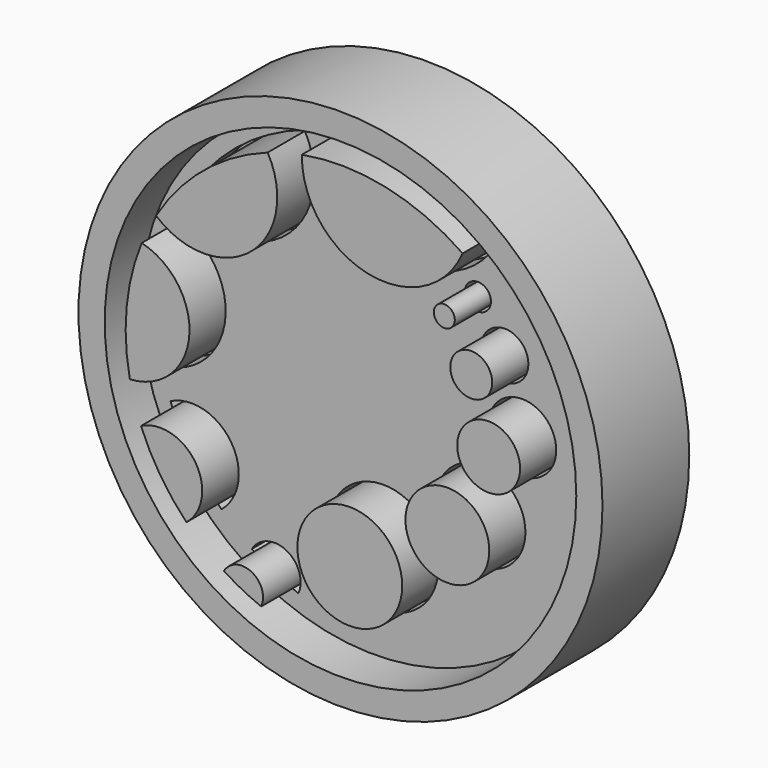
from build123d import *

# Parameters (mm, degrees)
F0_R         = 25
F0_R_2       = 22.5
F0_R_3       = 5
F0_R_4       = 4
F0_W         = 0.7168108311
F0_H         = 2.62805566
F0_R_5       = 2
F0_R_6       = 1
F0_R_7       = 3
F0_TEXT_SIZE = 4.8138397894
F2_DEPTH     = 4
F3_DEPTH     = 10.35
F4_DEPTH     = 10.35
F1_R         = 22.25
F1_R_2       = 5.25
F1_R_3       = 4.25
F1_W         = 0.7168108311
F1_H         = 2.62805566
F1_R_4       = 2.25
F1_R_5       = 1.25
F1_R_6       = 3.25
F1_TEXT_SIZE = 4.8138397894
F5_DEPTH     = 6.35


# Not quite as in the source:
# - Text() gives the source's letters only with a copy of the font that has no kerning and outlines rounded to 1/6400 em; it was checked with that copy


with BuildPart() as f2:
    # F0 (on Front) → F2 (new body)
    with BuildSketch(Plane.XZ):
        Circle(F0_R)
        Circle(F0_R_2, mode=Mode.SUBTRACT)
        Circle(F0_R_2)
        with BuildLine():
            ThreePointArc((11.6569283477, 16.8631557395), (18.1551236725, 9.5205821479), (20.5, 0))
            ThreePointArc((20.5, 0), (11.5132317321, -16.9615888136), (-7.5678531789, -19.0519709811))
            ThreePointArc((-7.5678531789, -19.0519709811), (-9.3883533238, -18.2238531016), (-11.1194937702, -17.2222779647))
            ThreePointArc((-11.1194937702, -17.2222779647), (-12.9920933667, -15.857348768), (-14.698689069, -14.2898054449))
            ThreePointArc((-14.698689069, -14.2898054449), (-17.1938340813, -11.1634255309), (-19.0343655416, -7.6120252515))
            ThreePointArc((-19.0343655416, -7.6120252515), (-19.6480708819, -5.8483596522), (-20.098740453, -4.0361655322))
            ThreePointArc((-20.098740453, -4.0361655322), (-20.406477126, 1.9559374492), (-18.9661277157, 7.7804883827))
            ThreePointArc((-18.9661277157, 7.7804883827), (-18.3325719196, 9.1742469344), (-17.5967657031, 10.5168358734))
            ThreePointArc((-17.5967657031, 10.5168358734), (-13.0325099947, 15.8241487366), (-6.9486992839, 19.2864091594))
            ThreePointArc((-6.9486992839, 19.2864091594), (-5.3345009161, 19.7937641689), (-3.6839600887, 20.1662698104))
            ThreePointArc((-3.6839600887, 20.1662698104), (4.315054618, 20.040716146), (11.6569283477, 16.8631557395))
        make_face(mode=Mode.SUBTRACT)
        with BuildLine():
            ThreePointArc((-7.5678531789, -19.0519709811), (11.5132317321, -16.9615888136), (20.5, 0))
            ThreePointArc((20.5, 0), (18.1551236725, 9.5205821479), (11.6569283477, 16.8631557395))
            ThreePointArc((11.6569283477, 16.8631557395), (2.6311308646, 12.2199488695), (-3.6839600887, 20.1662698104))
            ThreePointArc((-3.6839600887, 20.1662698104), (-5.3345009161, 19.7937641689), (-6.9486992839, 19.2864091594))
            ThreePointArc((-6.9486992839, 19.2864091594), (-8.5823846306, 10.4207808753), (-17.5967657031, 10.5168358734))
            ThreePointArc((-17.5967657031, 10.5168358734), (-18.3325719196, 9.1742469344), (-18.9661277157, 7.7804883827))
            ThreePointArc((-18.9661277157, 7.7804883827), (-14.4338496745, 1.3834679519), (-20.098740453, -4.0361655322))
            ThreePointArc((-20.098740453, -4.0361655322), (-19.6480708819, -5.8483596522), (-19.0343655416, -7.6120252515))
            ThreePointArc((-19.0343655416, -7.6120252515), (-13.8389396265, -8.985196159), (-14.698689069, -14.2898054449))
            ThreePointArc((-14.698689069, -14.2898054449), (-12.9920933667, -15.857348768), (-11.1194937702, -17.2222779647))
            ThreePointArc((-11.1194937702, -17.2222779647), (-8.4724164141, -16.4459162136), (-7.5678531789, -19.0519709811))
        make_face()
        with BuildLine():
            add(Edge.make_bspline(
                [(-3.0782241477, -4.3214418661), (-2.8995855618, -4.5527318248), (-2.8995855618, -4.8889484475)],
                knots=[0, 0, 0, 1, 1, 1], degree=2))
            add(Edge.make_bspline(
                [(-2.8995855618, -4.8889484475), (-2.8995855618, -5.3545370147), (-3.2346739408, -5.6226829342)],
                knots=[0, 0, 0, 1, 1, 1], degree=2))
            add(Edge.make_bspline(
                [(-3.2346739408, -5.6226829342), (-3.5697623199, -5.8908288537), (-4.1662271563, -5.8908288537)],
                knots=[0, 0, 0, 1, 1, 1], degree=2))
            add(Edge.make_bspline(
                [(-4.1662271563, -5.8908288537), (-4.7168100823, -5.8908288537), (-5.1395253888, -5.6832320128)],
                knots=[0, 0, 0, 1, 1, 1], degree=2))
            Line((-5.1395253888, -5.6832320128), (-5.1395253888, -5.0062857924))
            add(Edge.make_bspline(
                [(-5.1395253888, -5.0062857924), (-4.792026329, -5.1619834231), (-4.5509582583, -5.2251650703)],
                knots=[0, 0, 0, 1, 1, 1], degree=2))
            add(Edge.make_bspline(
                [(-4.5509582583, -5.2251650703), (-4.3098901876, -5.2883467176), (-4.1098149713, -5.2883467176)],
                knots=[0, 0, 0, 1, 1, 1], degree=2))
            add(Edge.make_bspline(
                [(-4.1098149713, -5.2883467176), (-3.8706273068, -5.2883467176), (-3.7423836061, -5.1969589778)],
                knots=[0, 0, 0, 1, 1, 1], degree=2))
            add(Edge.make_bspline(
                [(-3.7423836061, -5.1969589778), (-3.6141399055, -5.1055712381), (-3.6141399055, -4.9243000835)],
                knots=[0, 0, 0, 1, 1, 1], degree=2))
            add(Edge.make_bspline(
                [(-3.6141399055, -4.9243000835), (-3.6141399055, -4.8235103129), (-3.6705520905, -4.7445332539)],
                knots=[0, 0, 0, 1, 1, 1], degree=2))
            add(Edge.make_bspline(
                [(-3.6705520905, -4.7445332539), (-3.7269642756, -4.6655561948), (-3.8364039145, -4.5929725167)],
                knots=[0, 0, 0, 1, 1, 1], degree=2))
            add(Edge.make_bspline(
                [(-3.8364039145, -4.5929725167), (-3.9458435535, -4.5203888387), (-4.2820601763, -4.3601782332)],
                knots=[0, 0, 0, 1, 1, 1], degree=2))
            add(Edge.make_bspline(
                [(-4.2820601763, -4.3601782332), (-4.5964640875, -4.2120022272), (-4.7540421244, -4.0758608206)],
                knots=[0, 0, 0, 1, 1, 1], degree=2))
            add(Edge.make_bspline(
                [(-4.7540421244, -4.0758608206), (-4.9116201612, -3.9397194141), (-5.0056404696, -3.7584482595)],
                knots=[0, 0, 0, 1, 1, 1], degree=2))
            add(Edge.make_bspline(
                [(-5.0056404696, -3.7584482595), (-5.099660778, -3.5771771049), (-5.099660778, -3.335732953)],
                knots=[0, 0, 0, 1, 1, 1], degree=2))
            add(Edge.make_bspline(
                [(-5.099660778, -3.335732953), (-5.099660778, -2.8791703355), (-4.790522004, -2.6185460406)],
                knots=[0, 0, 0, 1, 1, 1], degree=2))
            add(Edge.make_bspline(
                [(-4.790522004, -2.6185460406), (-4.4813832301, -2.3579217458), (-3.9360654414, -2.3579217458)],
                knots=[0, 0, 0, 1, 1, 1], degree=2))
            add(Edge.make_bspline(
                [(-3.9360654414, -2.3579217458), (-3.6682956031, -2.3579217458), (-3.424971045, -2.421103393)],
                knots=[0, 0, 0, 1, 1, 1], degree=2))
            add(Edge.make_bspline(
                [(-3.424971045, -2.421103393), (-3.1816464869, -2.4842850402), (-2.916133136, -2.5993658977)],
                knots=[0, 0, 0, 1, 1, 1], degree=2))
            Line((-2.916133136, -2.5993658977), (-3.1508078258, -3.1664963979))
            add(Edge.make_bspline(
                [(-3.1508078258, -3.1664963979), (-3.4260992887, -3.0536720278), (-3.6058661184, -3.008918361)],
                knots=[0, 0, 0, 1, 1, 1], degree=2))
            add(Edge.make_bspline(
                [(-3.6058661184, -3.008918361), (-3.785632948, -2.9641646943), (-3.9593824779, -2.9641646943)],
                knots=[0, 0, 0, 1, 1, 1], degree=2))
            add(Edge.make_bspline(
                [(-3.9593824779, -2.9641646943), (-4.1662271563, -2.9641646943), (-4.276795039, -3.06044149)],
                knots=[0, 0, 0, 1, 1, 1], degree=2))
            add(Edge.make_bspline(
                [(-4.276795039, -3.06044149), (-4.3873629217, -3.1567182858), (-4.3873629217, -3.311663754)],
                knots=[0, 0, 0, 1, 1, 1], degree=2))
            add(Edge.make_bspline(
                [(-4.3873629217, -3.311663754), (-4.3873629217, -3.4079405498), (-4.3426092549, -3.4797720654)],
                knots=[0, 0, 0, 1, 1, 1], degree=2))
            add(Edge.make_bspline(
                [(-4.3426092549, -3.4797720654), (-4.2978555881, -3.5516035811), (-4.2004505486, -3.6185460406)],
                knots=[0, 0, 0, 1, 1, 1], degree=2))
            add(Edge.make_bspline(
                [(-4.2004505486, -3.6185460406), (-4.1030455091, -3.6854885002), (-3.738998875, -3.8592380301)],
                knots=[0, 0, 0, 1, 1, 1], degree=2))
            add(Edge.make_bspline(
                [(-3.738998875, -3.8592380301), (-3.2568627336, -4.0901519075), (-3.0782241477, -4.3214418661)],
                knots=[0, 0, 0, 1, 1, 1], degree=2))
        make_face(mode=Mode.SUBTRACT)
        with BuildLine():
            Line((-0.1541925569, -5.8434426183), (-0.8221128276, -5.8434426183))
            Line((-0.8221128276, -5.8434426183), (-1.6494915414, -3.1476923362))
            Line((-1.6494915414, -3.1476923362), (-1.6705520905, -3.1476923362))
            add(Edge.make_bspline(
                [(-1.6705520905, -3.1476923362), (-1.6254223425, -3.9698059128), (-1.6254223425, -4.2450973757)],
                knots=[0, 0, 0, 1, 1, 1], degree=2))
            Line((-1.6254223425, -4.2450973757), (-1.6254223425, -5.8434426183))
            Line((-1.6254223425, -5.8434426183), (-2.276795039, -5.8434426183))
            Line((-2.276795039, -5.8434426183), (-2.276795039, -2.4068123061))
            Line((-2.276795039, -2.4068123061), (-1.2846927449, -2.4068123061))
            Line((-1.2846927449, -2.4068123061), (-0.471605118, -5.0348679662))
            Line((-0.471605118, -5.0348679662), (-0.4573140311, -5.0348679662))
            Line((-0.4573140311, -5.0348679662), (0.4054163187, -2.4068123061))
            Line((0.4054163187, -2.4068123061), (1.3967664503, -2.4068123061))
            Line((1.3967664503, -2.4068123061), (1.3967664503, -5.8434426183))
            Line((1.3967664503, -5.8434426183), (0.7175637425, -5.8434426183))
            Line((0.7175637425, -5.8434426183), (0.7175637425, -4.216515202))
            add(Edge.make_bspline(
                [(0.7175637425, -4.216515202), (0.7175637425, -4.1014343445), (0.7213245548, -3.9510018511)],
                knots=[0, 0, 0, 1, 1, 1], degree=2))
            add(Edge.make_bspline(
                [(0.7213245548, -3.9510018511), (0.7250853672, -3.8005693577), (0.7529153784, -3.152205311)],
                knots=[0, 0, 0, 1, 1, 1], degree=2))
            Line((0.7529153784, -3.152205311), (0.7318548294, -3.152205311))
            Line((0.7318548294, -3.152205311), (-0.1541925569, -5.8434426183))
        make_face(mode=Mode.SUBTRACT)
        with Locations((0.8882983216, -12.9391586339)):
            Circle(F0_R_3, mode=Mode.SUBTRACT)
        with Locations((10.1970146039, -7.2864832287)):
            Circle(F0_R_4, mode=Mode.SUBTRACT)
        with BuildLine():
            Line((-9.9315524666, 0.7033794953), (-9.9315524666, 4.1400098074))
            Line((-9.9315524666, 4.1400098074), (-8.8619774384, 4.1400098074))
            add(Edge.make_bspline(
                [(-8.8619774384, 4.1400098074), (-8.1308755204, 4.1400098074), (-7.8006761973, 3.9320368853)],
                knots=[0, 0, 0, 1, 1, 1], degree=2))
            add(Edge.make_bspline(
                [(-7.8006761973, 3.9320368853), (-7.4704768743, 3.7240639631), (-7.4704768743, 3.2705099955)],
                knots=[0, 0, 0, 1, 1, 1], degree=2))
            add(Edge.make_bspline(
                [(-7.4704768743, 3.2705099955), (-7.4704768743, 2.962123384), (-7.614892068, 2.7646807364)],
                knots=[0, 0, 0, 1, 1, 1], degree=2))
            add(Edge.make_bspline(
                [(-7.614892068, 2.7646807364), (-7.7593072616, 2.5672380887), (-7.9992470886, 2.527373478)],
                knots=[0, 0, 0, 1, 1, 1], degree=2))
            Line((-7.9992470886, 2.527373478), (-7.9992470886, 2.5040564415))
            add(Edge.make_bspline(
                [(-7.9992470886, 2.5040564415), (-7.6728085779, 2.4310966822), (-7.528017303, 2.2313975472)],
                knots=[0, 0, 0, 1, 1, 1], degree=2))
            add(Edge.make_bspline(
                [(-7.528017303, 2.2313975472), (-7.3832260281, 2.0316984122), (-7.3832260281, 1.6999947642)],
                knots=[0, 0, 0, 1, 1, 1], degree=2))
            add(Edge.make_bspline(
                [(-7.3832260281, 1.6999947642), (-7.3832260281, 1.2298932223), (-7.7232034632, 0.9666363588)],
                knots=[0, 0, 0, 1, 1, 1], degree=2))
            add(Edge.make_bspline(
                [(-7.7232034632, 0.9666363588), (-8.0631808983, 0.7033794953), (-8.6461068103, 0.7033794953)],
                knots=[0, 0, 0, 1, 1, 1], degree=2))
            Line((-8.6461068103, 0.7033794953), (-9.9315524666, 0.7033794953))
        make_face(mode=Mode.SUBTRACT)
        with Locations((-6.3952606276, 2.0174073253)):
            Rectangle(F0_W, F0_H, mode=Mode.SUBTRACT)
        with BuildLine():
            add(Edge.make_bspline(
                [(-6.3941323839, 3.657873666), (-6.7845047043, 3.657873666), (-6.7845047043, 4.0106378631)],
                knots=[0, 0, 0, 1, 1, 1], degree=2))
            add(Edge.make_bspline(
                [(-6.7845047043, 4.0106378631), (-6.7845047043, 4.3611455728), (-6.3941323839, 4.3611455728)],
                knots=[0, 0, 0, 1, 1, 1], degree=2))
            add(Edge.make_bspline(
                [(-6.3941323839, 4.3611455728), (-6.0037600634, 4.3611455728), (-6.0037600634, 4.0106378631)],
                knots=[0, 0, 0, 1, 1, 1], degree=2))
            add(Edge.make_bspline(
                [(-6.0037600634, 4.0106378631), (-6.0037600634, 3.8436577954), (-6.1011651029, 3.7507657307)],
                knots=[0, 0, 0, 1, 1, 1], degree=2))
            add(Edge.make_bspline(
                [(-6.1011651029, 3.7507657307), (-6.1985701424, 3.657873666), (-6.3941323839, 3.657873666)],
                knots=[0, 0, 0, 1, 1, 1], degree=2))
        make_face(mode=Mode.SUBTRACT)
        with BuildLine():
            add(Edge.make_bspline(
                [(-3.0515223801, 2.7436201873), (-2.8965769119, 2.435609657), (-2.8965769119, 2.0219203001)],
                knots=[0, 0, 0, 1, 1, 1], degree=2))
            add(Edge.make_bspline(
                [(-2.8965769119, 2.0219203001), (-2.8965769119, 1.3803257157), (-3.2350500221, 1.0181594878)],
                knots=[0, 0, 0, 1, 1, 1], degree=2))
            add(Edge.make_bspline(
                [(-3.2350500221, 1.0181594878), (-3.5735231323, 0.6559932599), (-4.1775095933, 0.6559932599)],
                knots=[0, 0, 0, 1, 1, 1], degree=2))
            add(Edge.make_bspline(
                [(-4.1775095933, 0.6559932599), (-4.5558473143, 0.6559932599), (-4.8450537829, 0.8218450839)],
                knots=[0, 0, 0, 1, 1, 1], degree=2))
            add(Edge.make_bspline(
                [(-4.8450537829, 0.8218450839), (-5.1342602515, 0.9876969079), (-5.2892057197, 1.2979639255)],
                knots=[0, 0, 0, 1, 1, 1], degree=2))
            add(Edge.make_bspline(
                [(-5.2892057197, 1.2979639255), (-5.4441511879, 1.6082309432), (-5.4441511879, 2.0219203001)],
                knots=[0, 0, 0, 1, 1, 1], degree=2))
            add(Edge.make_bspline(
                [(-5.4441511879, 2.0219203001), (-5.4441511879, 2.6657713719), (-5.1083106464, 3.0230485438)],
                knots=[0, 0, 0, 1, 1, 1], degree=2))
            add(Edge.make_bspline(
                [(-5.1083106464, 3.0230485438), (-4.7724701048, 3.3803257157), (-4.1632185065, 3.3803257157)],
                knots=[0, 0, 0, 1, 1, 1], degree=2))
            add(Edge.make_bspline(
                [(-4.1632185065, 3.3803257157), (-3.7848807855, 3.3803257157), (-3.4956743169, 3.2159782166)],
                knots=[0, 0, 0, 1, 1, 1], degree=2))
            add(Edge.make_bspline(
                [(-3.4956743169, 3.2159782166), (-3.2064678483, 3.0516307176), (-3.0515223801, 2.7436201873)],
                knots=[0, 0, 0, 1, 1, 1], degree=2))
        make_face(mode=Mode.SUBTRACT)
        Polygon((-0.2685212519, 1.305109469), (-0.2685212519, 0.7033794953), (-2.2474607028, 0.7033794953), (-2.2474607028, 4.1400098074), (-0.2685212519, 4.1400098074), (-0.2685212519, 3.5427928086), (-1.5186152722, 3.5427928086), (-1.5186152722, 2.7883738541), (-0.3550199356, 2.7883738541), (-0.3550199356, 2.1911568552), (-1.5186152722, 2.1911568552), (-1.5186152722, 1.305109469), align=None, mode=Mode.SUBTRACT)
        with BuildLine():
            Line((3.2553599065, 4.1400098074), (3.2553599065, 0.7033794953))
            Line((3.2553599065, 0.7033794953), (2.5287709633, 0.7033794953))
            Line((2.5287709633, 0.7033794953), (2.5287709633, 2.6920970583))
            Line((2.5287709633, 2.6920970583), (2.5362925879, 3.018535569))
            Line((2.5362925879, 3.018535569), (2.5475750249, 3.3758127409))
            add(Edge.make_bspline(
                [(2.5475750249, 3.3758127409), (2.3670560328, 3.1952937488), (2.2963527609, 3.1388815637)],
                knots=[0, 0, 0, 1, 1, 1], degree=2))
            Line((2.2963527609, 3.1388815637), (1.9014674657, 2.8214690026))
            Line((1.9014674657, 2.8214690026), (1.550959756, 3.258475396))
            Line((1.550959756, 3.258475396), (2.6581429076, 4.1400098074))
            Line((2.6581429076, 4.1400098074), (3.2553599065, 4.1400098074))
        make_face(mode=Mode.SUBTRACT)
        with BuildLine():
            Line((6.6092523472, 1.314887581), (6.6092523472, 0.7033794953))
            Line((6.6092523472, 0.7033794953), (4.2068454273, 0.7033794953))
            Line((4.2068454273, 0.7033794953), (4.2068454273, 1.2088326732))
            Line((4.2068454273, 1.2088326732), (5.0695757771, 2.0805889725))
            add(Edge.make_bspline(
                [(5.0695757771, 2.0805889725), (5.4531786353, 2.4732177804), (5.5705159802, 2.6247785175)],
                knots=[0, 0, 0, 1, 1, 1], degree=2))
            add(Edge.make_bspline(
                [(5.5705159802, 2.6247785175), (5.687853325, 2.7763392546), (5.7397525353, 2.9057111989)],
                knots=[0, 0, 0, 1, 1, 1], degree=2))
            add(Edge.make_bspline(
                [(5.7397525353, 2.9057111989), (5.7916517455, 3.0350831433), (5.7916517455, 3.1734810372)],
                knots=[0, 0, 0, 1, 1, 1], degree=2))
            add(Edge.make_bspline(
                [(5.7916517455, 3.1734810372), (5.7916517455, 3.3803257157), (5.6773230505, 3.4814915675)],
                knots=[0, 0, 0, 1, 1, 1], degree=2))
            add(Edge.make_bspline(
                [(5.6773230505, 3.4814915675), (5.5629943555, 3.5826574193), (5.3726972513, 3.5826574193)],
                knots=[0, 0, 0, 1, 1, 1], degree=2))
            add(Edge.make_bspline(
                [(5.3726972513, 3.5826574193), (5.1733741976, 3.5826574193), (4.9853335808, 3.4908935983)],
                knots=[0, 0, 0, 1, 1, 1], degree=2))
            add(Edge.make_bspline(
                [(4.9853335808, 3.4908935983), (4.797292964, 3.3991297774), (4.592704773, 3.2298932223)],
                knots=[0, 0, 0, 1, 1, 1], degree=2))
            Line((4.592704773, 3.2298932223), (4.1978194777, 3.6977382768))
            add(Edge.make_bspline(
                [(4.1978194777, 3.6977382768), (4.4512982291, 3.9143610673), (4.6182782968, 4.0034923197)],
                knots=[0, 0, 0, 1, 1, 1], degree=2))
            add(Edge.make_bspline(
                [(4.6182782968, 4.0034923197), (4.7852583645, 4.092623572), (4.9827010121, 4.1407619699)],
                knots=[0, 0, 0, 1, 1, 1], degree=2))
            add(Edge.make_bspline(
                [(4.9827010121, 4.1407619699), (5.1801436598, 4.1889003678), (5.4245964616, 4.1889003678)],
                knots=[0, 0, 0, 1, 1, 1], degree=2))
            add(Edge.make_bspline(
                [(5.4245964616, 4.1889003678), (5.7465219975, 4.1889003678), (5.9932312867, 4.0715630229)],
                knots=[0, 0, 0, 1, 1, 1], degree=2))
            add(Edge.make_bspline(
                [(5.9932312867, 4.0715630229), (6.2399405759, 3.9542256781), (6.3764580637, 3.7424919436)],
                knots=[0, 0, 0, 1, 1, 1], degree=2))
            add(Edge.make_bspline(
                [(6.3764580637, 3.7424919436), (6.5129755514, 3.5307582091), (6.5129755514, 3.258475396)],
                knots=[0, 0, 0, 1, 1, 1], degree=2))
            add(Edge.make_bspline(
                [(6.5129755514, 3.258475396), (6.5129755514, 3.0207920564), (6.4294855176, 2.8128191343)],
                knots=[0, 0, 0, 1, 1, 1], degree=2))
            add(Edge.make_bspline(
                [(6.4294855176, 2.8128191343), (6.3459954838, 2.6048462121), (6.1707416289, 2.3863430154)],
                knots=[0, 0, 0, 1, 1, 1], degree=2))
            add(Edge.make_bspline(
                [(6.1707416289, 2.3863430154), (5.9954877741, 2.1678398187), (5.5539684059, 1.7631764114)],
                knots=[0, 0, 0, 1, 1, 1], degree=2))
            Line((5.5539684059, 1.7631764114), (5.1116968753, 1.3472305671))
            Line((5.1116968753, 1.3472305671), (5.1116968753, 1.314887581))
            Line((5.1116968753, 1.314887581), (6.6092523472, 1.314887581))
        make_face(mode=Mode.SUBTRACT)
        with BuildLine():
            add(Edge.make_bspline(
                [(8.9138781464, 3.9726536585), (9.2230169204, 3.7564069492), (9.2230169204, 3.3712997661)],
                knots=[0, 0, 0, 1, 1, 1], degree=2))
            add(Edge.make_bspline(
                [(9.2230169204, 3.3712997661), (9.2230169204, 3.0493742302), (9.0278307602, 2.82372549)],
                knots=[0, 0, 0, 1, 1, 1], degree=2))
            add(Edge.make_bspline(
                [(9.0278307602, 2.82372549), (8.8326446, 2.5980767499), (8.4798804029, 2.5130823911)],
                knots=[0, 0, 0, 1, 1, 1], degree=2))
            Line((8.4798804029, 2.5130823911), (8.4798804029, 2.4995434667))
            add(Edge.make_bspline(
                [(8.4798804029, 2.4995434667), (8.8965784097, 2.4476442565), (9.1101925503, 2.2464407965)],
                knots=[0, 0, 0, 1, 1, 1], degree=2))
            add(Edge.make_bspline(
                [(9.1101925503, 2.2464407965), (9.323806691, 2.0452373366), (9.323806691, 1.704507739)],
                knots=[0, 0, 0, 1, 1, 1], degree=2))
            add(Edge.make_bspline(
                [(9.323806691, 1.704507739), (9.323806691, 1.2088326732), (8.9642730317, 0.9324129665)],
                knots=[0, 0, 0, 1, 1, 1], degree=2))
            add(Edge.make_bspline(
                [(8.9642730317, 0.9324129665), (8.6047393724, 0.6559932599), (7.9375712641, 0.6559932599)],
                knots=[0, 0, 0, 1, 1, 1], degree=2))
            add(Edge.make_bspline(
                [(7.9375712641, 0.6559932599), (7.3779623886, 0.6559932599), (6.94546897, 0.8417773892)],
                knots=[0, 0, 0, 1, 1, 1], degree=2))
            Line((6.94546897, 0.8417773892), (6.94546897, 1.4600549372))
            add(Edge.make_bspline(
                [(6.94546897, 1.4600549372), (7.1447920238, 1.3592651666), (7.3847318508, 1.2957074381)],
                knots=[0, 0, 0, 1, 1, 1], degree=2))
            add(Edge.make_bspline(
                [(7.3847318508, 1.2957074381), (7.6246716778, 1.2321497097), (7.8593463675, 1.2321497097)],
                knots=[0, 0, 0, 1, 1, 1], degree=2))
            add(Edge.make_bspline(
                [(7.8593463675, 1.2321497097), (8.2196321893, 1.2321497097), (8.3911252318, 1.3543761106)],
                knots=[0, 0, 0, 1, 1, 1], degree=2))
            add(Edge.make_bspline(
                [(8.3911252318, 1.3543761106), (8.5626182743, 1.4766025115), (8.5626182743, 1.7473809996)],
                knots=[0, 0, 0, 1, 1, 1], degree=2))
            add(Edge.make_bspline(
                [(8.5626182743, 1.7473809996), (8.5626182743, 1.9888251516), (8.3651756267, 2.0899910034)],
                knots=[0, 0, 0, 1, 1, 1], degree=2))
            add(Edge.make_bspline(
                [(8.3651756267, 2.0899910034), (8.1677329791, 2.1911568552), (7.7352395605, 2.1911568552)],
                knots=[0, 0, 0, 1, 1, 1], degree=2))
            Line((7.7352395605, 2.1911568552), (7.4742391844, 2.1911568552))
            Line((7.4742391844, 2.1911568552), (7.4742391844, 2.7485092433))
            Line((7.4742391844, 2.7485092433), (7.7397525353, 2.7485092433))
            add(Edge.make_bspline(
                [(7.7397525353, 2.7485092433), (8.1391508053, 2.7485092433), (8.323806691, 2.8530598262)],
                knots=[0, 0, 0, 1, 1, 1], degree=2))
            add(Edge.make_bspline(
                [(8.323806691, 2.8530598262), (8.5084625766, 2.9576104092), (8.5084625766, 3.2110891606)],
                knots=[0, 0, 0, 1, 1, 1], degree=2))
            add(Edge.make_bspline(
                [(8.5084625766, 3.2110891606), (8.5084625766, 3.601461481), (8.019556973, 3.601461481)],
                knots=[0, 0, 0, 1, 1, 1], degree=2))
            add(Edge.make_bspline(
                [(8.019556973, 3.601461481), (7.8503204179, 3.601461481), (7.6750665631, 3.545049296)],
                knots=[0, 0, 0, 1, 1, 1], degree=2))
            add(Edge.make_bspline(
                [(7.6750665631, 3.545049296), (7.4998127083, 3.4886371109), (7.2861985676, 3.350239217)],
                knots=[0, 0, 0, 1, 1, 1], degree=2))
            Line((7.2861985676, 3.350239217), (6.9499819448, 3.8504272576))
            add(Edge.make_bspline(
                [(6.9499819448, 3.8504272576), (7.4200834868, 4.1889003678), (8.0714561833, 4.1889003678)],
                knots=[0, 0, 0, 1, 1, 1], degree=2))
            add(Edge.make_bspline(
                [(8.0714561833, 4.1889003678), (8.6047393724, 4.1889003678), (8.9138781464, 3.9726536585)],
                knots=[0, 0, 0, 1, 1, 1], degree=2))
        make_face(mode=Mode.SUBTRACT)
        with Locations((12.4771809766, 6.9347179564)):
            Circle(F0_R_5, mode=Mode.SUBTRACT)
        with Locations((9.9075548911, 11.027059711)):
            Circle(F0_R_6, mode=Mode.SUBTRACT)
        with Locations((14.1383596325, 0.5700431833)):
            Circle(F0_R_7, mode=Mode.SUBTRACT)
        with BuildLine():
            ThreePointArc((-3.6839600887, 20.1662698104), (2.6311308646, 12.2199488695), (11.6569283477, 16.8631557395))
            ThreePointArc((11.6569283477, 16.8631557395), (4.315054618, 20.040716146), (-3.6839600887, 20.1662698104))
        make_face()
        with Locations((0.8882983216, -12.9391586339)):
            Circle(F0_R_3)
        with BuildLine():
            ThreePointArc((-17.5967657031, 10.5168358734), (-8.5823846306, 10.4207808753), (-6.9486992839, 19.2864091594))
            ThreePointArc((-6.9486992839, 19.2864091594), (-13.0325099947, 15.8241487366), (-17.5967657031, 10.5168358734))
        make_face()
        with BuildLine():
            ThreePointArc((-20.098740453, -4.0361655322), (-14.4338496745, 1.3834679519), (-18.9661277157, 7.7804883827))
            ThreePointArc((-18.9661277157, 7.7804883827), (-20.406477126, 1.9559374492), (-20.098740453, -4.0361655322))
        make_face()
        with Locations((10.1970146039, -7.2864832287)):
            Circle(F0_R_4)
        with Locations((14.1383596325, 0.5700431833)):
            Circle(F0_R_7)
        with BuildLine():
            ThreePointArc((-19.0343655416, -7.6120252515), (-17.1938340813, -11.1634255309), (-14.698689069, -14.2898054449))
            ThreePointArc((-14.698689069, -14.2898054449), (-13.8389396265, -8.985196159), (-19.0343655416, -7.6120252515))
        make_face()
        with Locations((12.4771809766, 6.9347179564)):
            Circle(F0_R_5)
        with BuildLine():
            ThreePointArc((-11.1194937702, -17.2222779647), (-9.3883533238, -18.2238531016), (-7.5678531789, -19.0519709811))
            ThreePointArc((-7.5678531789, -19.0519709811), (-8.4724164141, -16.4459162136), (-11.1194937702, -17.2222779647))
        make_face()
        with Locations((-5.3606611541, -5.8434426183)):
            Text('SM', F0_TEXT_SIZE, font='Open Sans', font_style=FontStyle.BOLD, text_align=(TextAlign.LEFT, TextAlign.BOTTOM))
        with Locations((9.9075548911, 11.027059711)):
            Circle(F0_R_6)
        with BuildLine():
            add(Edge.make_bspline(
                [(-4.5866859754, 2.6086070244), (-4.7138014324, 2.4145491079), (-4.7138014324, 2.0219203001)],
                knots=[0, 0, 0, 1, 1, 1], degree=2))
            add(Edge.make_bspline(
                [(-4.7138014324, 2.0219203001), (-4.7138014324, 1.6315479797), (-4.5855577317, 1.4318488447)],
                knots=[0, 0, 0, 1, 1, 1], degree=2))
            add(Edge.make_bspline(
                [(-4.5855577317, 1.4318488447), (-4.4573140311, 1.2321497097), (-4.1684836437, 1.2321497097)],
                knots=[0, 0, 0, 1, 1, 1], degree=2))
            add(Edge.make_bspline(
                [(-4.1684836437, 1.2321497097), (-3.8811575813, 1.2321497097), (-3.7555464493, 1.430720601)],
                knots=[0, 0, 0, 1, 1, 1], degree=2))
            add(Edge.make_bspline(
                [(-3.7555464493, 1.430720601), (-3.6299353173, 1.6292914923), (-3.6299353173, 2.0219203001)],
                knots=[0, 0, 0, 1, 1, 1], degree=2))
            add(Edge.make_bspline(
                [(-3.6299353173, 2.0219203001), (-3.6299353173, 2.4122926205), (-3.756674693, 2.6074787807)],
                knots=[0, 0, 0, 1, 1, 1], degree=2))
            add(Edge.make_bspline(
                [(-3.756674693, 2.6074787807), (-3.8834140687, 2.8026649409), (-4.1729966185, 2.8026649409)],
                knots=[0, 0, 0, 1, 1, 1], degree=2))
            add(Edge.make_bspline(
                [(-4.1729966185, 2.8026649409), (-4.4595705185, 2.8026649409), (-4.5866859754, 2.6086070244)],
                knots=[0, 0, 0, 1, 1, 1], degree=2))
        make_face()
        with BuildLine():
            Line((-8.7514095557, 2.2009349673), (-9.202707036, 2.2009349673))
            Line((-9.202707036, 2.2009349673), (-9.202707036, 1.305109469))
            Line((-9.202707036, 1.305109469), (-8.7280925193, 1.305109469))
            add(Edge.make_bspline(
                [(-8.7280925193, 1.305109469), (-8.4272275324, 1.305109469), (-8.2839405824, 1.4201903264)],
                knots=[0, 0, 0, 1, 1, 1], degree=2))
            add(Edge.make_bspline(
                [(-8.2839405824, 1.4201903264), (-8.1406536325, 1.5352711839), (-8.1406536325, 1.7729545235)],
                knots=[0, 0, 0, 1, 1, 1], degree=2))
            add(Edge.make_bspline(
                [(-8.1406536325, 1.7729545235), (-8.1406536325, 2.2009349673), (-8.7514095557, 2.2009349673)],
                knots=[0, 0, 0, 1, 1, 1], degree=2))
        make_face()
        with BuildLine():
            Line((-9.202707036, 3.5427928086), (-9.202707036, 2.778595742))
            Line((-9.202707036, 2.778595742), (-8.7799917295, 2.778595742))
            add(Edge.make_bspline(
                [(-8.7799917295, 2.778595742), (-8.4836397175, 2.778595742), (-8.350883042, 2.870359563)],
                knots=[0, 0, 0, 1, 1, 1], degree=2))
            add(Edge.make_bspline(
                [(-8.350883042, 2.870359563), (-8.2181263666, 2.962123384), (-8.2181263666, 3.1734810372)],
                knots=[0, 0, 0, 1, 1, 1], degree=2))
            add(Edge.make_bspline(
                [(-8.2181263666, 3.1734810372), (-8.2181263666, 3.3712997661), (-8.3625415602, 3.4570462873)],
                knots=[0, 0, 0, 1, 1, 1], degree=2))
            add(Edge.make_bspline(
                [(-8.3625415602, 3.4570462873), (-8.5069567539, 3.5427928086), (-8.8198563402, 3.5427928086)],
                knots=[0, 0, 0, 1, 1, 1], degree=2))
            Line((-8.8198563402, 3.5427928086), (-9.202707036, 3.5427928086))
        make_face()
        with Locations((-10.3640458852, 0.7033794953)):
            Text('BioE 123', F0_TEXT_SIZE, font='Open Sans', font_style=FontStyle.BOLD, text_align=(TextAlign.LEFT, TextAlign.BOTTOM))
    extrude(amount=F2_DEPTH)

    # F0 (on Front) → F3 (join)
    with BuildSketch(Plane.XZ):
        Circle(F0_R)
        Circle(F0_R_2, mode=Mode.SUBTRACT)
    extrude(amount=F3_DEPTH)

    # F0 (on Front) → F4 (join, through all)
    with BuildSketch(Plane.XZ):
        with BuildLine():
            ThreePointArc((-11.1194937702, -17.2222779647), (-9.3883533238, -18.2238531016), (-7.5678531789, -19.0519709811))
            ThreePointArc((-7.5678531789, -19.0519709811), (-8.4724164141, -16.4459162136), (-11.1194937702, -17.2222779647))
        make_face()
        with BuildLine():
            ThreePointArc((-19.0343655416, -7.6120252515), (-17.1938340813, -11.1634255309), (-14.698689069, -14.2898054449))
            ThreePointArc((-14.698689069, -14.2898054449), (-13.8389396265, -8.985196159), (-19.0343655416, -7.6120252515))
        make_face()
        with BuildLine():
            ThreePointArc((-20.098740453, -4.0361655322), (-14.4338496745, 1.3834679519), (-18.9661277157, 7.7804883827))
            ThreePointArc((-18.9661277157, 7.7804883827), (-20.406477126, 1.9559374492), (-20.098740453, -4.0361655322))
        make_face()
        with BuildLine():
            ThreePointArc((-17.5967657031, 10.5168358734), (-8.5823846306, 10.4207808753), (-6.9486992839, 19.2864091594))
            ThreePointArc((-6.9486992839, 19.2864091594), (-13.0325099947, 15.8241487366), (-17.5967657031, 10.5168358734))
        make_face()
        with BuildLine():
            ThreePointArc((-3.6839600887, 20.1662698104), (2.6311308646, 12.2199488695), (11.6569283477, 16.8631557395))
            ThreePointArc((11.6569283477, 16.8631557395), (4.315054618, 20.040716146), (-3.6839600887, 20.1662698104))
        make_face()
        with Locations((9.9075548911, 11.027059711)):
            Circle(F0_R_6)
        with Locations((12.4771809766, 6.9347179564)):
            Circle(F0_R_5)
        with Locations((14.1383596325, 0.5700431833)):
            Circle(F0_R_7)
        with Locations((10.1970146039, -7.2864832287)):
            Circle(F0_R_4)
        with Locations((0.8882983216, -12.9391586339)):
            Circle(F0_R_3)
    extrude(amount=F4_DEPTH)


with BuildPart() as f5:
    # F1 (on Front) → F5 (new body)
    with BuildSketch(Plane.XZ):
        Circle(F1_R)
        with BuildLine():
            ThreePointArc((12.1346217877, 16.8319177181), (18.4710029789, 9.4543402177), (20.75, 0))
            ThreePointArc((20.75, 0), (11.8499176174, -17.0335537238), (-7.2154893938, -19.4550562273))
            ThreePointArc((-7.2154893938, -19.4550562273), (-9.5028454375, -18.4460952126), (-11.6522591755, -17.1693726183))
            ThreePointArc((-11.6522591755, -17.1693726183), (-13.1593057696, -16.0435398732), (-14.5581992197, -14.7858491633))
            ThreePointArc((-14.5581992197, -14.7858491633), (-17.4035149848, -11.2995648666), (-19.4303173437, -7.2818450907))
            ThreePointArc((-19.4303173437, -7.2818450907), (-19.8907911979, -5.9092237664), (-20.2544298794, -4.5078343204))
            ThreePointArc((-20.2544298794, -4.5078343204), (-20.6553366032, 1.979790345), (-19.0293878263, 8.2731432331))
            ThreePointArc((-19.0293878263, 8.2731432331), (-18.5537619442, 9.2908781994), (-18.0237538761, 10.281381046))
            ThreePointArc((-18.0237538761, 10.281381046), (-13.1914430434, 16.0171261602), (-6.6357618029, 19.6603449943))
            ThreePointArc((-6.6357618029, 19.6603449943), (-5.394509042, 20.0365109786), (-4.1321799146, 20.3343942411))
            ThreePointArc((-4.1321799146, 20.3343942411), (4.3676772353, 20.2851151234), (12.1346217877, 16.8319177181))
        make_face(mode=Mode.SUBTRACT)
        with BuildLine():
            ThreePointArc((-7.2154893938, -19.4550562273), (11.8499176174, -17.0335537238), (20.75, 0))
            ThreePointArc((20.75, 0), (18.4710029789, 9.4543402177), (12.1346217877, 16.8319177181))
            ThreePointArc((12.1346217877, 16.8319177181), (2.5785082473, 11.9755498921), (-4.1321799146, 20.3343942411))
            ThreePointArc((-4.1321799146, 20.3343942411), (-5.394509042, 20.0365109786), (-6.6357618029, 19.6603449943))
            ThreePointArc((-6.6357618029, 19.6603449943), (-8.4234515819, 10.2278034517), (-18.0237538761, 10.281381046))
            ThreePointArc((-18.0237538761, 10.281381046), (-18.5537619442, 9.2908781994), (-19.0293878263, 8.2731432331))
            ThreePointArc((-19.0293878263, 8.2731432331), (-14.1849901974, 1.3596150562), (-20.2544298794, -4.5078343204))
            ThreePointArc((-20.2544298794, -4.5078343204), (-19.8907911979, -5.9092237664), (-19.4303173437, -7.2818450907))
            ThreePointArc((-19.4303173437, -7.2818450907), (-13.629258723, -8.8490568232), (-14.5581992197, -14.7858491633))
            ThreePointArc((-14.5581992197, -14.7858491633), (-13.1593057696, -16.0435398732), (-11.6522591755, -17.1693726183))
            ThreePointArc((-11.6522591755, -17.1693726183), (-8.3579243004, -16.2236741026), (-7.2154893938, -19.4550562273))
        make_face()
        with BuildLine():
            add(Edge.make_bspline(
                [(-3.0782241477, -4.3214418661), (-2.8995855618, -4.5527318248), (-2.8995855618, -4.8889484475)],
                knots=[0, 0, 0, 1, 1, 1], degree=2))
            add(Edge.make_bspline(
                [(-2.8995855618, -4.8889484475), (-2.8995855618, -5.3545370147), (-3.2346739408, -5.6226829342)],
                knots=[0, 0, 0, 1, 1, 1], degree=2))
            add(Edge.make_bspline(
                [(-3.2346739408, -5.6226829342), (-3.5697623199, -5.8908288537), (-4.1662271563, -5.8908288537)],
                knots=[0, 0, 0, 1, 1, 1], degree=2))
            add(Edge.make_bspline(
                [(-4.1662271563, -5.8908288537), (-4.7168100823, -5.8908288537), (-5.1395253888, -5.6832320128)],
                knots=[0, 0, 0, 1, 1, 1], degree=2))
            Line((-5.1395253888, -5.6832320128), (-5.1395253888, -5.0062857924))
            add(Edge.make_bspline(
                [(-5.1395253888, -5.0062857924), (-4.792026329, -5.1619834231), (-4.5509582583, -5.2251650703)],
                knots=[0, 0, 0, 1, 1, 1], degree=2))
            add(Edge.make_bspline(
                [(-4.5509582583, -5.2251650703), (-4.3098901876, -5.2883467176), (-4.1098149713, -5.2883467176)],
                knots=[0, 0, 0, 1, 1, 1], degree=2))
            add(Edge.make_bspline(
                [(-4.1098149713, -5.2883467176), (-3.8706273068, -5.2883467176), (-3.7423836061, -5.1969589778)],
                knots=[0, 0, 0, 1, 1, 1], degree=2))
            add(Edge.make_bspline(
                [(-3.7423836061, -5.1969589778), (-3.6141399055, -5.1055712381), (-3.6141399055, -4.9243000835)],
                knots=[0, 0, 0, 1, 1, 1], degree=2))
            add(Edge.make_bspline(
                [(-3.6141399055, -4.9243000835), (-3.6141399055, -4.8235103129), (-3.6705520905, -4.7445332539)],
                knots=[0, 0, 0, 1, 1, 1], degree=2))
            add(Edge.make_bspline(
                [(-3.6705520905, -4.7445332539), (-3.7269642756, -4.6655561948), (-3.8364039145, -4.5929725167)],
                knots=[0, 0, 0, 1, 1, 1], degree=2))
            add(Edge.make_bspline(
                [(-3.8364039145, -4.5929725167), (-3.9458435535, -4.5203888387), (-4.2820601763, -4.3601782332)],
                knots=[0, 0, 0, 1, 1, 1], degree=2))
            add(Edge.make_bspline(
                [(-4.2820601763, -4.3601782332), (-4.5964640875, -4.2120022272), (-4.7540421244, -4.0758608206)],
                knots=[0, 0, 0, 1, 1, 1], degree=2))
            add(Edge.make_bspline(
                [(-4.7540421244, -4.0758608206), (-4.9116201612, -3.9397194141), (-5.0056404696, -3.7584482595)],
                knots=[0, 0, 0, 1, 1, 1], degree=2))
            add(Edge.make_bspline(
                [(-5.0056404696, -3.7584482595), (-5.099660778, -3.5771771049), (-5.099660778, -3.335732953)],
                knots=[0, 0, 0, 1, 1, 1], degree=2))
            add(Edge.make_bspline(
                [(-5.099660778, -3.335732953), (-5.099660778, -2.8791703355), (-4.790522004, -2.6185460406)],
                knots=[0, 0, 0, 1, 1, 1], degree=2))
            add(Edge.make_bspline(
                [(-4.790522004, -2.6185460406), (-4.4813832301, -2.3579217458), (-3.9360654414, -2.3579217458)],
                knots=[0, 0, 0, 1, 1, 1], degree=2))
            add(Edge.make_bspline(
                [(-3.9360654414, -2.3579217458), (-3.6682956031, -2.3579217458), (-3.424971045, -2.421103393)],
                knots=[0, 0, 0, 1, 1, 1], degree=2))
            add(Edge.make_bspline(
                [(-3.424971045, -2.421103393), (-3.1816464869, -2.4842850402), (-2.916133136, -2.5993658977)],
                knots=[0, 0, 0, 1, 1, 1], degree=2))
            Line((-2.916133136, -2.5993658977), (-3.1508078258, -3.1664963979))
            add(Edge.make_bspline(
                [(-3.1508078258, -3.1664963979), (-3.4260992887, -3.0536720278), (-3.6058661184, -3.008918361)],
                knots=[0, 0, 0, 1, 1, 1], degree=2))
            add(Edge.make_bspline(
                [(-3.6058661184, -3.008918361), (-3.785632948, -2.9641646943), (-3.9593824779, -2.9641646943)],
                knots=[0, 0, 0, 1, 1, 1], degree=2))
            add(Edge.make_bspline(
                [(-3.9593824779, -2.9641646943), (-4.1662271563, -2.9641646943), (-4.276795039, -3.06044149)],
                knots=[0, 0, 0, 1, 1, 1], degree=2))
            add(Edge.make_bspline(
                [(-4.276795039, -3.06044149), (-4.3873629217, -3.1567182858), (-4.3873629217, -3.311663754)],
                knots=[0, 0, 0, 1, 1, 1], degree=2))
            add(Edge.make_bspline(
                [(-4.3873629217, -3.311663754), (-4.3873629217, -3.4079405498), (-4.3426092549, -3.4797720654)],
                knots=[0, 0, 0, 1, 1, 1], degree=2))
            add(Edge.make_bspline(
                [(-4.3426092549, -3.4797720654), (-4.2978555881, -3.5516035811), (-4.2004505486, -3.6185460406)],
                knots=[0, 0, 0, 1, 1, 1], degree=2))
            add(Edge.make_bspline(
                [(-4.2004505486, -3.6185460406), (-4.1030455091, -3.6854885002), (-3.738998875, -3.8592380301)],
                knots=[0, 0, 0, 1, 1, 1], degree=2))
            add(Edge.make_bspline(
                [(-3.738998875, -3.8592380301), (-3.2568627336, -4.0901519075), (-3.0782241477, -4.3214418661)],
                knots=[0, 0, 0, 1, 1, 1], degree=2))
        make_face(mode=Mode.SUBTRACT)
        with BuildLine():
            Line((-0.1541925569, -5.8434426183), (-0.8221128276, -5.8434426183))
            Line((-0.8221128276, -5.8434426183), (-1.6494915414, -3.1476923362))
            Line((-1.6494915414, -3.1476923362), (-1.6705520905, -3.1476923362))
            add(Edge.make_bspline(
                [(-1.6705520905, -3.1476923362), (-1.6254223425, -3.9698059128), (-1.6254223425, -4.2450973757)],
                knots=[0, 0, 0, 1, 1, 1], degree=2))
            Line((-1.6254223425, -4.2450973757), (-1.6254223425, -5.8434426183))
            Line((-1.6254223425, -5.8434426183), (-2.276795039, -5.8434426183))
            Line((-2.276795039, -5.8434426183), (-2.276795039, -2.4068123061))
            Line((-2.276795039, -2.4068123061), (-1.2846927449, -2.4068123061))
            Line((-1.2846927449, -2.4068123061), (-0.471605118, -5.0348679662))
            Line((-0.471605118, -5.0348679662), (-0.4573140311, -5.0348679662))
            Line((-0.4573140311, -5.0348679662), (0.4054163187, -2.4068123061))
            Line((0.4054163187, -2.4068123061), (1.3967664503, -2.4068123061))
            Line((1.3967664503, -2.4068123061), (1.3967664503, -5.8434426183))
            Line((1.3967664503, -5.8434426183), (0.7175637425, -5.8434426183))
            Line((0.7175637425, -5.8434426183), (0.7175637425, -4.216515202))
            add(Edge.make_bspline(
                [(0.7175637425, -4.216515202), (0.7175637425, -4.1014343445), (0.7213245548, -3.9510018511)],
                knots=[0, 0, 0, 1, 1, 1], degree=2))
            add(Edge.make_bspline(
                [(0.7213245548, -3.9510018511), (0.7250853672, -3.8005693577), (0.7529153784, -3.152205311)],
                knots=[0, 0, 0, 1, 1, 1], degree=2))
            Line((0.7529153784, -3.152205311), (0.7318548294, -3.152205311))
            Line((0.7318548294, -3.152205311), (-0.1541925569, -5.8434426183))
        make_face(mode=Mode.SUBTRACT)
        with Locations((0.8882983216, -12.9391586339)):
            Circle(F1_R_2, mode=Mode.SUBTRACT)
        with Locations((10.1970146039, -7.2864832287)):
            Circle(F1_R_3, mode=Mode.SUBTRACT)
        with BuildLine():
            Line((-9.9315524666, 0.7033794953), (-9.9315524666, 4.1400098074))
            Line((-9.9315524666, 4.1400098074), (-8.8619774384, 4.1400098074))
            add(Edge.make_bspline(
                [(-8.8619774384, 4.1400098074), (-8.1308755204, 4.1400098074), (-7.8006761973, 3.9320368853)],
                knots=[0, 0, 0, 1, 1, 1], degree=2))
            add(Edge.make_bspline(
                [(-7.8006761973, 3.9320368853), (-7.4704768743, 3.7240639631), (-7.4704768743, 3.2705099955)],
                knots=[0, 0, 0, 1, 1, 1], degree=2))
            add(Edge.make_bspline(
                [(-7.4704768743, 3.2705099955), (-7.4704768743, 2.962123384), (-7.614892068, 2.7646807364)],
                knots=[0, 0, 0, 1, 1, 1], degree=2))
            add(Edge.make_bspline(
                [(-7.614892068, 2.7646807364), (-7.7593072616, 2.5672380887), (-7.9992470886, 2.527373478)],
                knots=[0, 0, 0, 1, 1, 1], degree=2))
            Line((-7.9992470886, 2.527373478), (-7.9992470886, 2.5040564415))
            add(Edge.make_bspline(
                [(-7.9992470886, 2.5040564415), (-7.6728085779, 2.4310966822), (-7.528017303, 2.2313975472)],
                knots=[0, 0, 0, 1, 1, 1], degree=2))
            add(Edge.make_bspline(
                [(-7.528017303, 2.2313975472), (-7.3832260281, 2.0316984122), (-7.3832260281, 1.6999947642)],
                knots=[0, 0, 0, 1, 1, 1], degree=2))
            add(Edge.make_bspline(
                [(-7.3832260281, 1.6999947642), (-7.3832260281, 1.2298932223), (-7.7232034632, 0.9666363588)],
                knots=[0, 0, 0, 1, 1, 1], degree=2))
            add(Edge.make_bspline(
                [(-7.7232034632, 0.9666363588), (-8.0631808983, 0.7033794953), (-8.6461068103, 0.7033794953)],
                knots=[0, 0, 0, 1, 1, 1], degree=2))
            Line((-8.6461068103, 0.7033794953), (-9.9315524666, 0.7033794953))
        make_face(mode=Mode.SUBTRACT)
        with Locations((-6.3952606276, 2.0174073253)):
            Rectangle(F1_W, F1_H, mode=Mode.SUBTRACT)
        with BuildLine():
            add(Edge.make_bspline(
                [(-6.3941323839, 3.657873666), (-6.7845047043, 3.657873666), (-6.7845047043, 4.0106378631)],
                knots=[0, 0, 0, 1, 1, 1], degree=2))
            add(Edge.make_bspline(
                [(-6.7845047043, 4.0106378631), (-6.7845047043, 4.3611455728), (-6.3941323839, 4.3611455728)],
                knots=[0, 0, 0, 1, 1, 1], degree=2))
            add(Edge.make_bspline(
                [(-6.3941323839, 4.3611455728), (-6.0037600634, 4.3611455728), (-6.0037600634, 4.0106378631)],
                knots=[0, 0, 0, 1, 1, 1], degree=2))
            add(Edge.make_bspline(
                [(-6.0037600634, 4.0106378631), (-6.0037600634, 3.8436577954), (-6.1011651029, 3.7507657307)],
                knots=[0, 0, 0, 1, 1, 1], degree=2))
            add(Edge.make_bspline(
                [(-6.1011651029, 3.7507657307), (-6.1985701424, 3.657873666), (-6.3941323839, 3.657873666)],
                knots=[0, 0, 0, 1, 1, 1], degree=2))
        make_face(mode=Mode.SUBTRACT)
        with BuildLine():
            add(Edge.make_bspline(
                [(-3.0515223801, 2.7436201873), (-2.8965769119, 2.435609657), (-2.8965769119, 2.0219203001)],
                knots=[0, 0, 0, 1, 1, 1], degree=2))
            add(Edge.make_bspline(
                [(-2.8965769119, 2.0219203001), (-2.8965769119, 1.3803257157), (-3.2350500221, 1.0181594878)],
                knots=[0, 0, 0, 1, 1, 1], degree=2))
            add(Edge.make_bspline(
                [(-3.2350500221, 1.0181594878), (-3.5735231323, 0.6559932599), (-4.1775095933, 0.6559932599)],
                knots=[0, 0, 0, 1, 1, 1], degree=2))
            add(Edge.make_bspline(
                [(-4.1775095933, 0.6559932599), (-4.5558473143, 0.6559932599), (-4.8450537829, 0.8218450839)],
                knots=[0, 0, 0, 1, 1, 1], degree=2))
            add(Edge.make_bspline(
                [(-4.8450537829, 0.8218450839), (-5.1342602515, 0.9876969079), (-5.2892057197, 1.2979639255)],
                knots=[0, 0, 0, 1, 1, 1], degree=2))
            add(Edge.make_bspline(
                [(-5.2892057197, 1.2979639255), (-5.4441511879, 1.6082309432), (-5.4441511879, 2.0219203001)],
                knots=[0, 0, 0, 1, 1, 1], degree=2))
            add(Edge.make_bspline(
                [(-5.4441511879, 2.0219203001), (-5.4441511879, 2.6657713719), (-5.1083106464, 3.0230485438)],
                knots=[0, 0, 0, 1, 1, 1], degree=2))
            add(Edge.make_bspline(
                [(-5.1083106464, 3.0230485438), (-4.7724701048, 3.3803257157), (-4.1632185065, 3.3803257157)],
                knots=[0, 0, 0, 1, 1, 1], degree=2))
            add(Edge.make_bspline(
                [(-4.1632185065, 3.3803257157), (-3.7848807855, 3.3803257157), (-3.4956743169, 3.2159782166)],
                knots=[0, 0, 0, 1, 1, 1], degree=2))
            add(Edge.make_bspline(
                [(-3.4956743169, 3.2159782166), (-3.2064678483, 3.0516307176), (-3.0515223801, 2.7436201873)],
                knots=[0, 0, 0, 1, 1, 1], degree=2))
        make_face(mode=Mode.SUBTRACT)
        Polygon((-0.2685212519, 1.305109469), (-0.2685212519, 0.7033794953), (-2.2474607028, 0.7033794953), (-2.2474607028, 4.1400098074), (-0.2685212519, 4.1400098074), (-0.2685212519, 3.5427928086), (-1.5186152722, 3.5427928086), (-1.5186152722, 2.7883738541), (-0.3550199356, 2.7883738541), (-0.3550199356, 2.1911568552), (-1.5186152722, 2.1911568552), (-1.5186152722, 1.305109469), align=None, mode=Mode.SUBTRACT)
        with BuildLine():
            Line((3.2553599065, 4.1400098074), (3.2553599065, 0.7033794953))
            Line((3.2553599065, 0.7033794953), (2.5287709633, 0.7033794953))
            Line((2.5287709633, 0.7033794953), (2.5287709633, 2.6920970583))
            Line((2.5287709633, 2.6920970583), (2.5362925879, 3.018535569))
            Line((2.5362925879, 3.018535569), (2.5475750249, 3.3758127409))
            add(Edge.make_bspline(
                [(2.5475750249, 3.3758127409), (2.3670560328, 3.1952937488), (2.2963527609, 3.1388815637)],
                knots=[0, 0, 0, 1, 1, 1], degree=2))
            Line((2.2963527609, 3.1388815637), (1.9014674657, 2.8214690026))
            Line((1.9014674657, 2.8214690026), (1.550959756, 3.258475396))
            Line((1.550959756, 3.258475396), (2.6581429076, 4.1400098074))
            Line((2.6581429076, 4.1400098074), (3.2553599065, 4.1400098074))
        make_face(mode=Mode.SUBTRACT)
        with BuildLine():
            Line((6.6092523472, 1.314887581), (6.6092523472, 0.7033794953))
            Line((6.6092523472, 0.7033794953), (4.2068454273, 0.7033794953))
            Line((4.2068454273, 0.7033794953), (4.2068454273, 1.2088326732))
            Line((4.2068454273, 1.2088326732), (5.0695757771, 2.0805889725))
            add(Edge.make_bspline(
                [(5.0695757771, 2.0805889725), (5.4531786353, 2.4732177804), (5.5705159802, 2.6247785175)],
                knots=[0, 0, 0, 1, 1, 1], degree=2))
            add(Edge.make_bspline(
                [(5.5705159802, 2.6247785175), (5.687853325, 2.7763392546), (5.7397525353, 2.9057111989)],
                knots=[0, 0, 0, 1, 1, 1], degree=2))
            add(Edge.make_bspline(
                [(5.7397525353, 2.9057111989), (5.7916517455, 3.0350831433), (5.7916517455, 3.1734810372)],
                knots=[0, 0, 0, 1, 1, 1], degree=2))
            add(Edge.make_bspline(
                [(5.7916517455, 3.1734810372), (5.7916517455, 3.3803257157), (5.6773230505, 3.4814915675)],
                knots=[0, 0, 0, 1, 1, 1], degree=2))
            add(Edge.make_bspline(
                [(5.6773230505, 3.4814915675), (5.5629943555, 3.5826574193), (5.3726972513, 3.5826574193)],
                knots=[0, 0, 0, 1, 1, 1], degree=2))
            add(Edge.make_bspline(
                [(5.3726972513, 3.5826574193), (5.1733741976, 3.5826574193), (4.9853335808, 3.4908935983)],
                knots=[0, 0, 0, 1, 1, 1], degree=2))
            add(Edge.make_bspline(
                [(4.9853335808, 3.4908935983), (4.797292964, 3.3991297774), (4.592704773, 3.2298932223)],
                knots=[0, 0, 0, 1, 1, 1], degree=2))
            Line((4.592704773, 3.2298932223), (4.1978194777, 3.6977382768))
            add(Edge.make_bspline(
                [(4.1978194777, 3.6977382768), (4.4512982291, 3.9143610673), (4.6182782968, 4.0034923197)],
                knots=[0, 0, 0, 1, 1, 1], degree=2))
            add(Edge.make_bspline(
                [(4.6182782968, 4.0034923197), (4.7852583645, 4.092623572), (4.9827010121, 4.1407619699)],
                knots=[0, 0, 0, 1, 1, 1], degree=2))
            add(Edge.make_bspline(
                [(4.9827010121, 4.1407619699), (5.1801436598, 4.1889003678), (5.4245964616, 4.1889003678)],
                knots=[0, 0, 0, 1, 1, 1], degree=2))
            add(Edge.make_bspline(
                [(5.4245964616, 4.1889003678), (5.7465219975, 4.1889003678), (5.9932312867, 4.0715630229)],
                knots=[0, 0, 0, 1, 1, 1], degree=2))
            add(Edge.make_bspline(
                [(5.9932312867, 4.0715630229), (6.2399405759, 3.9542256781), (6.3764580637, 3.7424919436)],
                knots=[0, 0, 0, 1, 1, 1], degree=2))
            add(Edge.make_bspline(
                [(6.3764580637, 3.7424919436), (6.5129755514, 3.5307582091), (6.5129755514, 3.258475396)],
                knots=[0, 0, 0, 1, 1, 1], degree=2))
            add(Edge.make_bspline(
                [(6.5129755514, 3.258475396), (6.5129755514, 3.0207920564), (6.4294855176, 2.8128191343)],
                knots=[0, 0, 0, 1, 1, 1], degree=2))
            add(Edge.make_bspline(
                [(6.4294855176, 2.8128191343), (6.3459954838, 2.6048462121), (6.1707416289, 2.3863430154)],
                knots=[0, 0, 0, 1, 1, 1], degree=2))
            add(Edge.make_bspline(
                [(6.1707416289, 2.3863430154), (5.9954877741, 2.1678398187), (5.5539684059, 1.7631764114)],
                knots=[0, 0, 0, 1, 1, 1], degree=2))
            Line((5.5539684059, 1.7631764114), (5.1116968753, 1.3472305671))
            Line((5.1116968753, 1.3472305671), (5.1116968753, 1.314887581))
            Line((5.1116968753, 1.314887581), (6.6092523472, 1.314887581))
        make_face(mode=Mode.SUBTRACT)
        with BuildLine():
            add(Edge.make_bspline(
                [(8.9138781464, 3.9726536585), (9.2230169204, 3.7564069492), (9.2230169204, 3.3712997661)],
                knots=[0, 0, 0, 1, 1, 1], degree=2))
            add(Edge.make_bspline(
                [(9.2230169204, 3.3712997661), (9.2230169204, 3.0493742302), (9.0278307602, 2.82372549)],
                knots=[0, 0, 0, 1, 1, 1], degree=2))
            add(Edge.make_bspline(
                [(9.0278307602, 2.82372549), (8.8326446, 2.5980767499), (8.4798804029, 2.5130823911)],
                knots=[0, 0, 0, 1, 1, 1], degree=2))
            Line((8.4798804029, 2.5130823911), (8.4798804029, 2.4995434667))
            add(Edge.make_bspline(
                [(8.4798804029, 2.4995434667), (8.8965784097, 2.4476442565), (9.1101925503, 2.2464407965)],
                knots=[0, 0, 0, 1, 1, 1], degree=2))
            add(Edge.make_bspline(
                [(9.1101925503, 2.2464407965), (9.323806691, 2.0452373366), (9.323806691, 1.704507739)],
                knots=[0, 0, 0, 1, 1, 1], degree=2))
            add(Edge.make_bspline(
                [(9.323806691, 1.704507739), (9.323806691, 1.2088326732), (8.9642730317, 0.9324129665)],
                knots=[0, 0, 0, 1, 1, 1], degree=2))
            add(Edge.make_bspline(
                [(8.9642730317, 0.9324129665), (8.6047393724, 0.6559932599), (7.9375712641, 0.6559932599)],
                knots=[0, 0, 0, 1, 1, 1], degree=2))
            add(Edge.make_bspline(
                [(7.9375712641, 0.6559932599), (7.3779623886, 0.6559932599), (6.94546897, 0.8417773892)],
                knots=[0, 0, 0, 1, 1, 1], degree=2))
            Line((6.94546897, 0.8417773892), (6.94546897, 1.4600549372))
            add(Edge.make_bspline(
                [(6.94546897, 1.4600549372), (7.1447920238, 1.3592651666), (7.3847318508, 1.2957074381)],
                knots=[0, 0, 0, 1, 1, 1], degree=2))
            add(Edge.make_bspline(
                [(7.3847318508, 1.2957074381), (7.6246716778, 1.2321497097), (7.8593463675, 1.2321497097)],
                knots=[0, 0, 0, 1, 1, 1], degree=2))
            add(Edge.make_bspline(
                [(7.8593463675, 1.2321497097), (8.2196321893, 1.2321497097), (8.3911252318, 1.3543761106)],
                knots=[0, 0, 0, 1, 1, 1], degree=2))
            add(Edge.make_bspline(
                [(8.3911252318, 1.3543761106), (8.5626182743, 1.4766025115), (8.5626182743, 1.7473809996)],
                knots=[0, 0, 0, 1, 1, 1], degree=2))
            add(Edge.make_bspline(
                [(8.5626182743, 1.7473809996), (8.5626182743, 1.9888251516), (8.3651756267, 2.0899910034)],
                knots=[0, 0, 0, 1, 1, 1], degree=2))
            add(Edge.make_bspline(
                [(8.3651756267, 2.0899910034), (8.1677329791, 2.1911568552), (7.7352395605, 2.1911568552)],
                knots=[0, 0, 0, 1, 1, 1], degree=2))
            Line((7.7352395605, 2.1911568552), (7.4742391844, 2.1911568552))
            Line((7.4742391844, 2.1911568552), (7.4742391844, 2.7485092433))
            Line((7.4742391844, 2.7485092433), (7.7397525353, 2.7485092433))
            add(Edge.make_bspline(
                [(7.7397525353, 2.7485092433), (8.1391508053, 2.7485092433), (8.323806691, 2.8530598262)],
                knots=[0, 0, 0, 1, 1, 1], degree=2))
            add(Edge.make_bspline(
                [(8.323806691, 2.8530598262), (8.5084625766, 2.9576104092), (8.5084625766, 3.2110891606)],
                knots=[0, 0, 0, 1, 1, 1], degree=2))
            add(Edge.make_bspline(
                [(8.5084625766, 3.2110891606), (8.5084625766, 3.601461481), (8.019556973, 3.601461481)],
                knots=[0, 0, 0, 1, 1, 1], degree=2))
            add(Edge.make_bspline(
                [(8.019556973, 3.601461481), (7.8503204179, 3.601461481), (7.6750665631, 3.545049296)],
                knots=[0, 0, 0, 1, 1, 1], degree=2))
            add(Edge.make_bspline(
                [(7.6750665631, 3.545049296), (7.4998127083, 3.4886371109), (7.2861985676, 3.350239217)],
                knots=[0, 0, 0, 1, 1, 1], degree=2))
            Line((7.2861985676, 3.350239217), (6.9499819448, 3.8504272576))
            add(Edge.make_bspline(
                [(6.9499819448, 3.8504272576), (7.4200834868, 4.1889003678), (8.0714561833, 4.1889003678)],
                knots=[0, 0, 0, 1, 1, 1], degree=2))
            add(Edge.make_bspline(
                [(8.0714561833, 4.1889003678), (8.6047393724, 4.1889003678), (8.9138781464, 3.9726536585)],
                knots=[0, 0, 0, 1, 1, 1], degree=2))
        make_face(mode=Mode.SUBTRACT)
        with Locations((12.4771809766, 6.9347179564)):
            Circle(F1_R_4, mode=Mode.SUBTRACT)
        with Locations((9.9075548911, 11.027059711)):
            Circle(F1_R_5, mode=Mode.SUBTRACT)
        with Locations((14.1383596325, 0.5700431833)):
            Circle(F1_R_6, mode=Mode.SUBTRACT)
        with Locations((-5.3606611541, -5.8434426183)):
            Text('SM', F1_TEXT_SIZE, font='Open Sans', font_style=FontStyle.BOLD, text_align=(TextAlign.LEFT, TextAlign.BOTTOM))
        with BuildLine():
            add(Edge.make_bspline(
                [(-4.5866859754, 2.6086070244), (-4.7138014324, 2.4145491079), (-4.7138014324, 2.0219203001)],
                knots=[0, 0, 0, 1, 1, 1], degree=2))
            add(Edge.make_bspline(
                [(-4.7138014324, 2.0219203001), (-4.7138014324, 1.6315479797), (-4.5855577317, 1.4318488447)],
                knots=[0, 0, 0, 1, 1, 1], degree=2))
            add(Edge.make_bspline(
                [(-4.5855577317, 1.4318488447), (-4.4573140311, 1.2321497097), (-4.1684836437, 1.2321497097)],
                knots=[0, 0, 0, 1, 1, 1], degree=2))
            add(Edge.make_bspline(
                [(-4.1684836437, 1.2321497097), (-3.8811575813, 1.2321497097), (-3.7555464493, 1.430720601)],
                knots=[0, 0, 0, 1, 1, 1], degree=2))
            add(Edge.make_bspline(
                [(-3.7555464493, 1.430720601), (-3.6299353173, 1.6292914923), (-3.6299353173, 2.0219203001)],
                knots=[0, 0, 0, 1, 1, 1], degree=2))
            add(Edge.make_bspline(
                [(-3.6299353173, 2.0219203001), (-3.6299353173, 2.4122926205), (-3.756674693, 2.6074787807)],
                knots=[0, 0, 0, 1, 1, 1], degree=2))
            add(Edge.make_bspline(
                [(-3.756674693, 2.6074787807), (-3.8834140687, 2.8026649409), (-4.1729966185, 2.8026649409)],
                knots=[0, 0, 0, 1, 1, 1], degree=2))
            add(Edge.make_bspline(
                [(-4.1729966185, 2.8026649409), (-4.4595705185, 2.8026649409), (-4.5866859754, 2.6086070244)],
                knots=[0, 0, 0, 1, 1, 1], degree=2))
        make_face()
        with BuildLine():
            Line((-8.7514095557, 2.2009349673), (-9.202707036, 2.2009349673))
            Line((-9.202707036, 2.2009349673), (-9.202707036, 1.305109469))
            Line((-9.202707036, 1.305109469), (-8.7280925193, 1.305109469))
            add(Edge.make_bspline(
                [(-8.7280925193, 1.305109469), (-8.4272275324, 1.305109469), (-8.2839405824, 1.4201903264)],
                knots=[0, 0, 0, 1, 1, 1], degree=2))
            add(Edge.make_bspline(
                [(-8.2839405824, 1.4201903264), (-8.1406536325, 1.5352711839), (-8.1406536325, 1.7729545235)],
                knots=[0, 0, 0, 1, 1, 1], degree=2))
            add(Edge.make_bspline(
                [(-8.1406536325, 1.7729545235), (-8.1406536325, 2.2009349673), (-8.7514095557, 2.2009349673)],
                knots=[0, 0, 0, 1, 1, 1], degree=2))
        make_face()
        with BuildLine():
            Line((-9.202707036, 3.5427928086), (-9.202707036, 2.778595742))
            Line((-9.202707036, 2.778595742), (-8.7799917295, 2.778595742))
            add(Edge.make_bspline(
                [(-8.7799917295, 2.778595742), (-8.4836397175, 2.778595742), (-8.350883042, 2.870359563)],
                knots=[0, 0, 0, 1, 1, 1], degree=2))
            add(Edge.make_bspline(
                [(-8.350883042, 2.870359563), (-8.2181263666, 2.962123384), (-8.2181263666, 3.1734810372)],
                knots=[0, 0, 0, 1, 1, 1], degree=2))
            add(Edge.make_bspline(
                [(-8.2181263666, 3.1734810372), (-8.2181263666, 3.3712997661), (-8.3625415602, 3.4570462873)],
                knots=[0, 0, 0, 1, 1, 1], degree=2))
            add(Edge.make_bspline(
                [(-8.3625415602, 3.4570462873), (-8.5069567539, 3.5427928086), (-8.8198563402, 3.5427928086)],
                knots=[0, 0, 0, 1, 1, 1], degree=2))
            Line((-8.8198563402, 3.5427928086), (-9.202707036, 3.5427928086))
        make_face()
        with Locations((-10.3640458852, 0.7033794953)):
            Text('BioE 123', F1_TEXT_SIZE, font='Open Sans', font_style=FontStyle.BOLD, text_align=(TextAlign.LEFT, TextAlign.BOTTOM))
    extrude(amount=F5_DEPTH)


solid = Compound([f2.part, f5.part])
